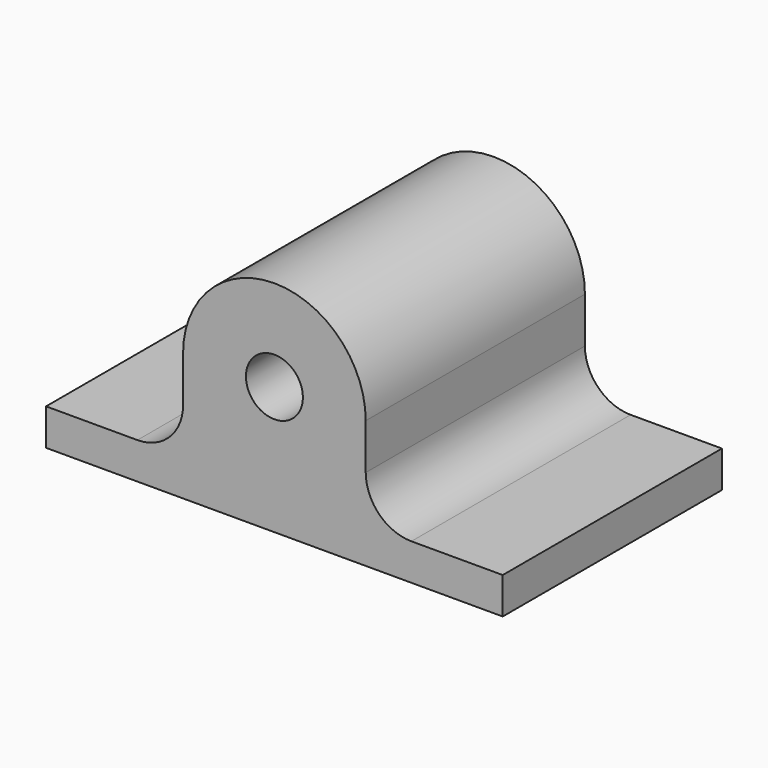
from build123d import *

# Parameters (mm, degrees)
F1_DEPTH = 76.2
F2_R     = 12.7
F3_R     = 7.921290647
F4_DEPTH = 101.6


# Not quite as in the source:
# - a feature names something its author has since deleted; it is built from what else it names


with BuildPart() as f1:
    # F0 (on Front) → F1 (new body)
    with BuildSketch(Plane.XZ):
        with BuildLine():
            Line((25.4, -25.4), (25.4, 0))
            ThreePointArc((25.4, 0), (0, 25.4), (-25.4, 0))
            Line((-25.4, 0), (-25.4, -25.4))
            Line((-25.4, -25.4), (-63.5, -25.4))
            Line((-63.5, -25.4), (-63.5, -35.56))
            Line((-63.5, -35.56), (63.5, -35.56))
            Line((63.5, -35.56), (63.5, -25.4))
            Line((63.5, -25.4), (25.4, -25.4))
        make_face()
    extrude(amount=F1_DEPTH)

    # F2
    f2_edges = [f1.edges().sort_by_distance(p)[0] for p in [
        (25.4, -38.1, -25.4),
        (-25.4, -38.1, -25.4),
    ]]
    fillet(f2_edges, radius=F2_R)

    # F3 (on face) → F4 (cut)
    with BuildSketch(Plane.XZ.offset(76.2)):
        Circle(F3_R)
    extrude(amount=-F4_DEPTH, mode=Mode.SUBTRACT)


solid = f1.part
